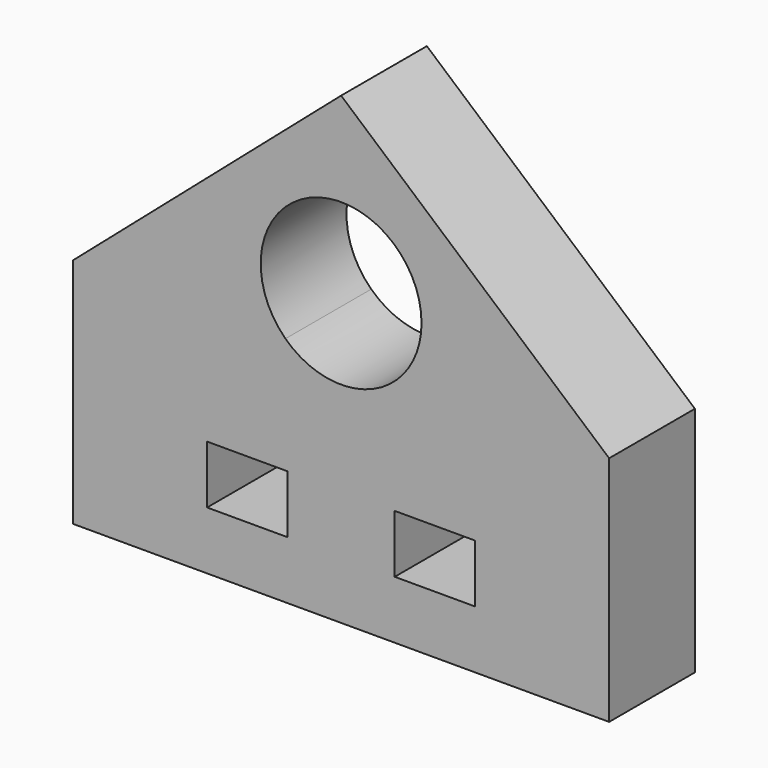
from build123d import *

# Parameters (mm, degrees)
F1_DEPTH = 6.35


# Not quite as in the source:
# - a feature names something its author has since deleted; it is built from what else it names


with BuildPart() as f1:
    # F0 (on Front) → F1 (new body)
    with BuildSketch(Plane.XZ):
        Polygon((1.984375, 3.4370383213), (0, 0), (7.9375, 0), (15.875, 0), (31.75, 0), (29.765625, 3.4370383213), (23.8125, 3.4370383213), (19.05, 3.4370383213), (15.875, 3.4370383213), (12.7, 3.4370383213), (11.90625, 3.4370383213), (7.9375, 3.4370383213), align=None)
        Polygon((0, 3.4370383213), (0, 0), (1.984375, 3.4370383213), align=None)
        Polygon((0, 3.4370383213), (1.984375, 3.4370383213), (7.9375, 13.7481532851), (0, 13.7481532851), (0, 6.8740766425), align=None)
        with BuildLine():
            Line((7.9375, 13.7481532851), (1.984375, 3.4370383213))
            Line((1.984375, 3.4370383213), (7.9375, 3.4370383213))
            Line((7.9375, 3.4370383213), (7.9375, 6.8740766425))
            Line((7.9375, 6.8740766425), (12.7, 6.8740766425))
            Line((12.7, 6.8740766425), (15.875, 6.8740766425))
            Line((15.875, 6.8740766425), (19.05, 6.8740766425))
            Line((19.05, 6.8740766425), (23.8125, 6.8740766425))
            Line((23.8125, 6.8740766425), (23.8125, 3.4370383213))
            Line((23.8125, 3.4370383213), (29.765625, 3.4370383213))
            Line((29.765625, 3.4370383213), (23.8125, 13.7481532851))
            Line((23.8125, 13.7481532851), (19.1716913456, 13.7481532851))
            ThreePointArc((19.1716913456, 13.7481532851), (15.875, 12.4226916063), (12.5783086544, 13.7481532851))
            Line((12.5783086544, 13.7481532851), (7.9375, 13.7481532851))
        make_face()
        Polygon((0, 13.7481532851), (7.9375, 13.7481532851), (15.875, 27.4963065702), align=None)
        with BuildLine():
            Line((15.875, 27.4963065702), (7.9375, 13.7481532851))
            Line((7.9375, 13.7481532851), (12.5783086544, 13.7481532851))
            ThreePointArc((12.5783086544, 13.7481532851), (14.0067235595, 21.56593919), (20.6375, 17.1851916063))
            ThreePointArc((20.6375, 17.1851916063), (20.2557475837, 15.3169151658), (19.1716913456, 13.7481532851))
            Line((19.1716913456, 13.7481532851), (23.8125, 13.7481532851))
            Line((23.8125, 13.7481532851), (15.875, 27.4963065702))
        make_face()
        Polygon((29.765625, 3.4370383213), (31.75, 0), (31.75, 3.4370383213), align=None)
        Polygon((31.75, 13.7481532851), (15.875, 27.4963065702), (23.8125, 13.7481532851), align=None)
        Polygon((23.8125, 13.7481532851), (29.765625, 3.4370383213), (31.75, 3.4370383213), (31.75, 13.7481532851), align=None)
        Polygon((12.7, 6.8740766425), (12.7, 3.4370383213), (15.875, 3.4370383213), (19.05, 3.4370383213), (19.05, 6.8740766425), (15.875, 6.8740766425), align=None)
    extrude(amount=F1_DEPTH)


solid = f1.part
